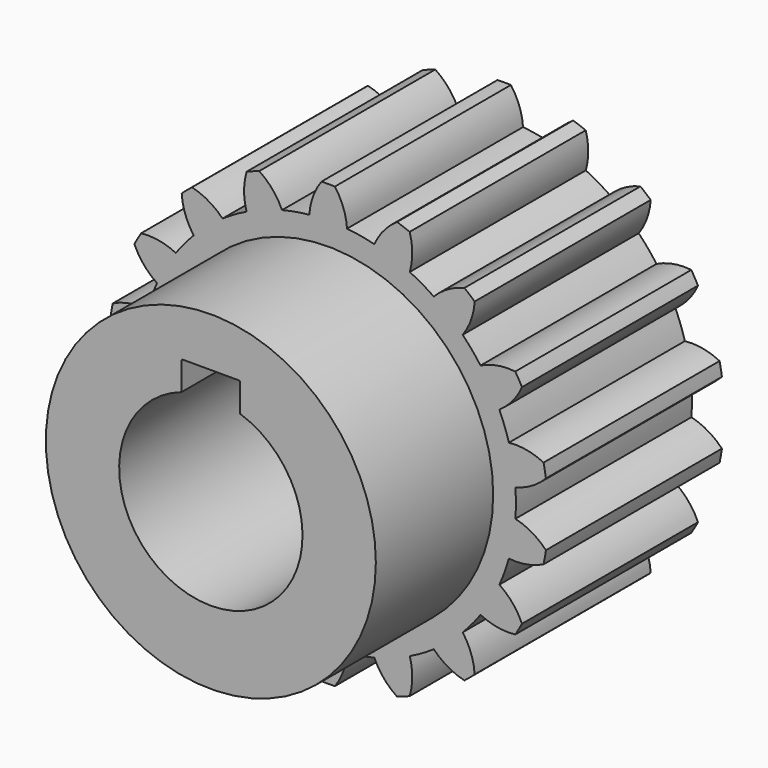
from build123d import *

# Parameters (mm, degrees)
F0_R     = 25.6
F1_DEPTH = 30
F3_DEPTH = 30
F4_COUNT = 18
F5_R     = 22.5
F6_DEPTH = 20
F8_DEPTH = 50.001
F9_R     = 0.2


with BuildPart() as f1:
    # F0 (on Front) → F1 (new body)
    with BuildSketch(Plane.XZ):
        Circle(F0_R)
    extrude(amount=F1_DEPTH)

    # F2 (on Front) → F3 (join, through all)
    with BuildSketch(Plane.XZ):
        with BuildLine():
            ThreePointArc((-2.5717175805, 25.4704980062), (0, 25.6), (2.5717175805, 25.4704980062))
            ThreePointArc((2.5717175805, 25.4704980062), (2.0656887709, 27.8468218747), (0.9139195769, 29.9860759521))
            ThreePointArc((0.9139195769, 29.9860759521), (0, 30), (-0.9139195769, 29.9860759521))
            ThreePointArc((-0.9139195769, 29.9860759521), (-2.0656887709, 27.8468218747), (-2.5717175805, 25.4704980062))
        make_face()
    extrude(amount=F3_DEPTH)

    # F4: F1 ×18 about axis
    f4_axis = Axis((0, 0, 0), (0, 1, 0))


with BuildPart() as f1_1:
    add(f1.part)
    for i in range(1, F4_COUNT):
        add(f1.part.rotate(f4_axis, i * 360 / F4_COUNT))

    # F5 (on face) → F6 (join)
    with BuildSketch(Plane.XZ.offset(30)):
        Circle(F5_R)
    extrude(amount=F6_DEPTH)

    # F7 (on Front) → F8 (cut, through all)
    with BuildSketch(Plane.XZ):
        with BuildLine():
            Line((4, 15.8), (-4, 15.8))
            Line((-4, 15.8), (-4, 11.8427192823))
            ThreePointArc((-4, 11.8427192823), (0, -12.5), (4, 11.8427192823))
            Line((4, 11.8427192823), (4, 15.8))
        make_face()
    extrude(amount=F8_DEPTH, mode=Mode.SUBTRACT)

    # F9
    f9_edges = [f1_1.edges().sort_by_distance(p)[0] for p in [
        (-4, -25, 15.8),
        (4, -25, 15.8),
    ]]
    fillet(f9_edges, radius=F9_R)


solid = f1_1.part
